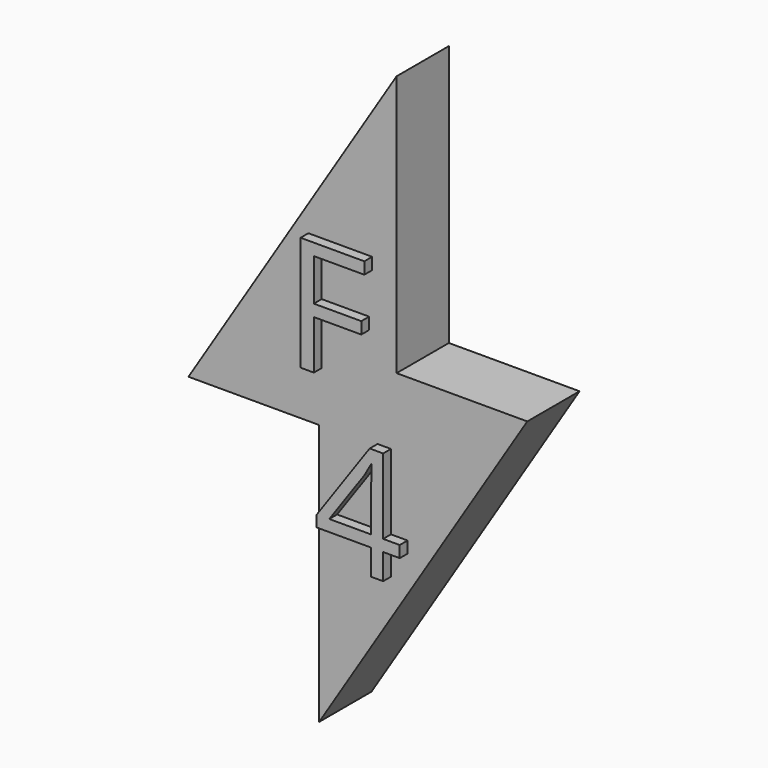
from build123d import *

# Parameters (mm, degrees)
F1_DEPTH     = 12.7
F2_TEXT_SIZE = 31.142422534
F4_DEPTH     = 1.905
F3_TEXT_SIZE = 30.458964304
F5_DEPTH     = 1.905


# Not quite as in the source:
# - Text() gives the source's letters only with a copy of the font that has no kerning and outlines rounded to 1/6400 em; it was checked with that copy


with BuildPart() as f1:
    # F0 (on Front) → F1 (new body)
    with BuildSketch(Plane.XZ):
        Polygon((29.9722214752, -5.4223644547), (29.9722214752, 45.3776355453), (-10.4832379147, -19.1963205481), (14.9167620853, -19.1963205481), (14.9167620853, -69.9963205481), (55.3722214752, -5.4223644547), align=None)
    extrude(amount=F1_DEPTH)

    # F2 (on face) → F4 (join)
    with BuildSketch(Plane.XZ.offset(12.7)):
        with Locations((9.7722979058, -9.2875033087)):
            Text('F', F2_TEXT_SIZE, font='Open Sans', text_align=(TextAlign.LEFT, TextAlign.BOTTOM))
    extrude(amount=F4_DEPTH)

    # F3 (on face) → F5 (join)
    with BuildSketch(Plane.XZ.offset(12.7)):
        with Locations((15.3031181544, -40.6074896455)):
            Text('4', F3_TEXT_SIZE, font='Open Sans', text_align=(TextAlign.LEFT, TextAlign.BOTTOM))
    extrude(amount=F5_DEPTH)


solid = f1.part
